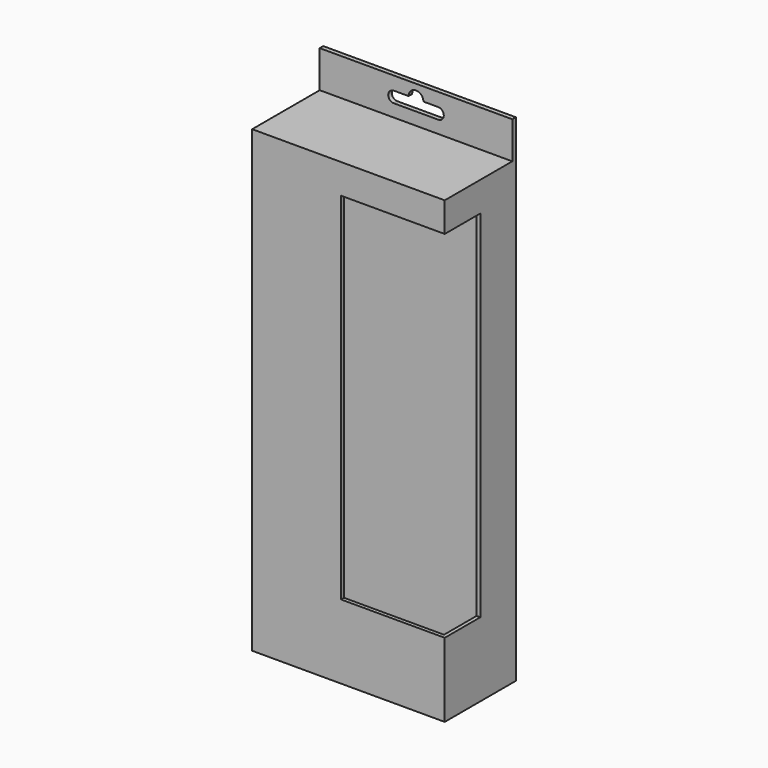
from build123d import *

# Parameters (mm, degrees)
F0_W      = 130
F0_H      = 310
F1_DEPTH  = 60
F3_DEPTH  = 30
F4_T      = -2.5
F5_W      = 130
F5_H      = 3
F6_DEPTH  = 25
F10_DEPTH = 3.001
F11_DEPTH = 25
F12_DEPTH = 3.001


# Not quite as in the source:
# - a feature of the source that left no trace in its solid (it failed there, or was rolled back) is left out


with BuildPart() as f1:
    # F0 (on Front) → F1 (new body)
    with BuildSketch(Plane.XZ):
        with Locations((-65, 155)):
            Rectangle(F0_W, F0_H)
    extrude(amount=F1_DEPTH)

    # F2 (on face) → F3 (cut)
    with BuildSketch(Plane.XZ.offset(60)):
        Polygon((0, 50), (0, 290), (-70, 290), (-70, 50), (-48.1321327388, 50), align=None)
    extrude(amount=-F3_DEPTH, mode=Mode.SUBTRACT)

    # F4
    f4_openings = [f1.faces().sort_by_distance(p)[0] for p in [
        (-35, -45, 50),
        (-70, -45, 170),
        (-35, -30, 170),
        (-35, -45, 290),
    ]]
    offset(amount=F4_T, openings=f4_openings)

    # F5 (on face) → F6 (join)
    with BuildSketch(Plane.XY.offset(310)):
        with Locations((-65, -1.5)):
            Rectangle(F5_W, F5_H)
    extrude(amount=F6_DEPTH)

    # F9 (on face) → F10 (cut, through all)
    with BuildSketch(Plane.XZ.offset(3)):
        with BuildLine():
            Line((-50, 326), (-60, 326))
            ThreePointArc((-60, 326), (-65, 331), (-70, 326))
            Line((-70, 326), (-80, 326))
            ThreePointArc((-80, 326), (-83.75, 322.25), (-80, 318.5))
            Line((-80, 318.5), (-50, 318.5))
            ThreePointArc((-50, 318.5), (-46.25, 322.25), (-50, 326))
        make_face()
    extrude(amount=-F10_DEPTH, mode=Mode.SUBTRACT)

    # F5 (on face) → F11 (join)
    with BuildSketch(Plane.XY.offset(310)):
        with Locations((-65, -1.5)):
            Rectangle(F5_W, F5_H)
    extrude(amount=F11_DEPTH)

    # F9 (on face) → F12 (cut, through all)
    with BuildSketch(Plane.XZ.offset(3)):
        with BuildLine():
            Line((-50, 326), (-60, 326))
            ThreePointArc((-60, 326), (-65, 331), (-70, 326))
            Line((-70, 326), (-80, 326))
            ThreePointArc((-80, 326), (-83.75, 322.25), (-80, 318.5))
            Line((-80, 318.5), (-50, 318.5))
            ThreePointArc((-50, 318.5), (-46.25, 322.25), (-50, 326))
        make_face()
    extrude(amount=-F12_DEPTH, mode=Mode.SUBTRACT)


solid = f1.part
